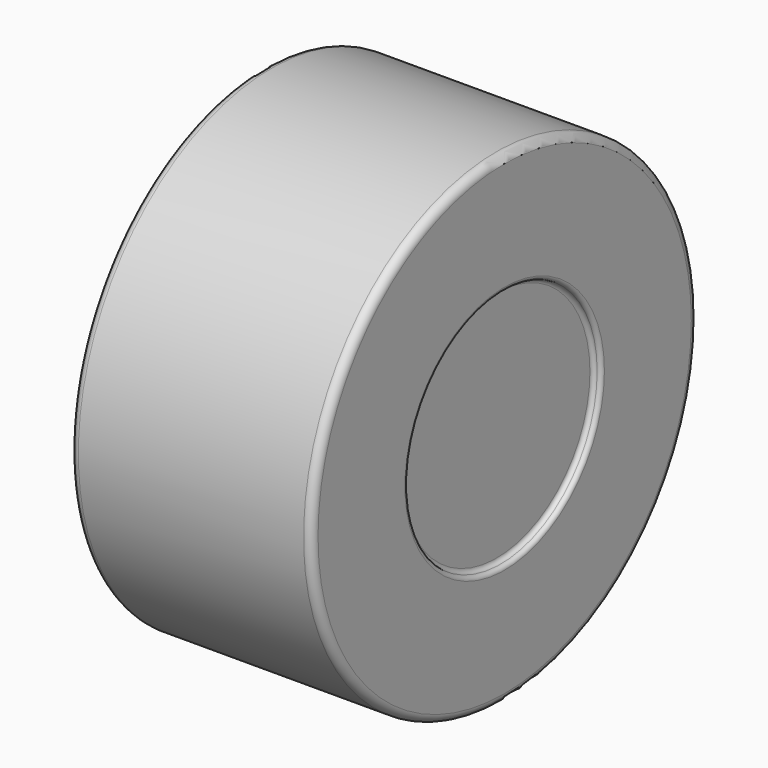
from build123d import *

# Parameters (mm, degrees)
F0_R      = 75
F1_DEPTH  = 75
F2_R      = 55
F3_DEPTH  = 40
F4_R      = 37.5
F5_DEPTH  = 30
F6_R      = 10
F7_DEPTH  = 30
F8_R      = 2.5
F9_R      = 37.5
F10_DEPTH = 2.5
F11_R     = 1.24999
F12_R     = 5


# Not quite as in the source:
# - a fillet or chamfer is up to 0.001 mm smaller than in the source, because OpenCascade refuses the exact size


with BuildPart() as f1:
    # F0 (on Right) → F1 (new body)
    with BuildSketch(Plane.YZ):
        Circle(F0_R)
    extrude(amount=F1_DEPTH)

    # F2 (on face) → F3 (cut)
    with BuildSketch(Plane(origin=(0, 0, 0), x_dir=(0, -1, 0), z_dir=(-1, 0, 0))):
        Circle(F2_R)
    extrude(amount=-F3_DEPTH, mode=Mode.SUBTRACT)

    # F4 (on face) → F5 (join)
    with BuildSketch(Plane(origin=(40, 0, 0), x_dir=(0, -1, 0), z_dir=(-1, 0, 0))):
        Circle(F4_R)
    extrude(amount=F5_DEPTH)

    # F6 (on face) → F7 (cut)
    with BuildSketch(Plane(origin=(10, 0, 0), x_dir=(0, -1, 0), z_dir=(-1, 0, 0))):
        Circle(F6_R)
    extrude(amount=-F7_DEPTH, mode=Mode.SUBTRACT)

    # F8
    f8_edges = [f1.edges().sort_by_distance(p)[0] for p in [
        (40, 37.5, 0),
        (37.5, 75, 0),
        (0, -75, 0),
        (75, -75, 0),
    ]]
    fillet(f8_edges, radius=F8_R)

    # F9 (on face) → F10 (cut)
    with BuildSketch(Plane.YZ.offset(75)):
        Circle(F9_R)
    extrude(amount=-F10_DEPTH, mode=Mode.SUBTRACT)

    # F11 (radius 1.25 in the source; OpenCascade refuses exactly that, so slightly less here)
    f11_edges = [f1.edges().sort_by_distance(p)[0] for p in [
        (72.5, -37.5, 0),
        (75, -37.5, 0),
    ]]
    fillet(f11_edges, radius=F11_R)

    # F12
    f12_edges = [f1.edges().sort_by_distance(p)[0] for p in [
        (40, 55, 0),
    ]]
    fillet(f12_edges, radius=F12_R)


solid = f1.part
